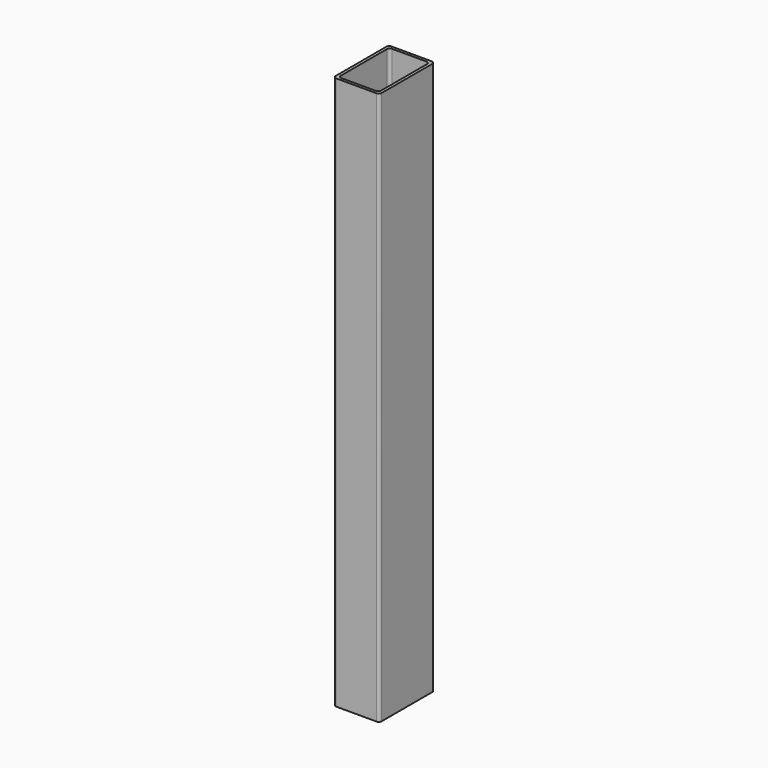
from build123d import *

# Parameters (mm, degrees)
F0_W     = 50.8
F0_H     = 76.2
F0_W_2   = 44.45
F0_H_2   = 69.85
F2_DEPTH = 609.6
F3_R     = 3.175


# Not quite as in the source:
# - a variable given as a bare number and used for a length is read in inches; the dataset says mm whatever the document's units were


with BuildPart() as f2:
    # F0 (on Top) → F2 (new body)
    with BuildSketch(Plane.XY):
        Rectangle(F0_W, F0_H)
        Rectangle(F0_W_2, F0_H_2, mode=Mode.SUBTRACT)
    extrude(amount=F2_DEPTH)

    # F3
    f3_edges = [f2.edges().sort_by_distance(p)[0] for p in [
        (-22.225, 34.925, 304.8),
        (22.225, 34.925, 304.8),
        (22.225, -34.925, 304.8),
        (-22.225, -34.925, 304.8),
        (25.4, 38.1, 304.8),
        (-25.4, 38.1, 304.8),
        (25.4, -38.1, 304.8),
        (-25.4, -38.1, 304.8),
    ]]
    fillet(f3_edges, radius=F3_R)


solid = f2.part
